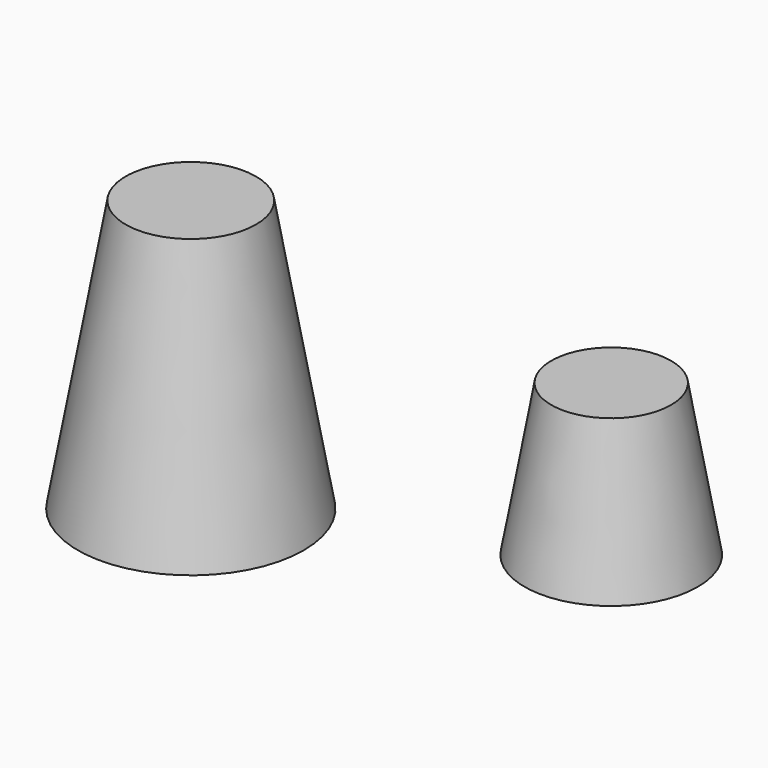
from build123d import *

# Parameters (mm, degrees)
F0_R     = 38.5091671968
F1_DEPTH = 67
F3_R     = 50
F4_DEPTH = 120
F4_TAPER = 10


# Not quite as in the source:
# - a fillet or chamfer that OpenCascade refuses, or shapes differently, is made with other operations: its cross-section is extruded or revolved along the edge and cut away or added


with BuildPart() as f1:
    # F0 (on Top) → F1 (new body)
    with BuildSketch(Plane.XY):
        Circle(F0_R)
    extrude(amount=F1_DEPTH)

    # F2: chamfer of 12 x 68.0553818354 on 1 edges, made by hand

    # F2_s1 → F2_t2 (revolve, cut)
    with BuildSketch(Plane.XZ):
        Polygon((38.5091671968, -1.0553818354), (26.5091671968, 67), (38.5091671968, 67), align=None)
    revolve(axis=Axis((0, 0, 67), (0, 0, 1)), mode=Mode.SUBTRACT)


with BuildPart() as f4:
    # F3 (on Top) → F4 (new body)
    with BuildSketch(Plane.XY):
        with Locations((-135.0683420897, -63.6841207743)):
            Circle(F3_R)
    extrude(amount=F4_DEPTH, taper=F4_TAPER)


solid = Compound([f1.part, f4.part])
